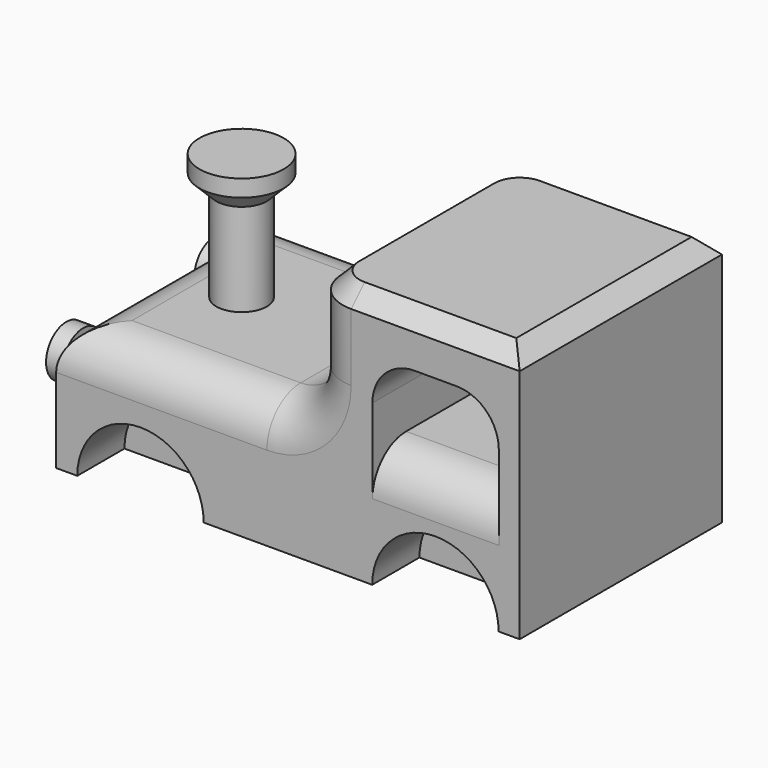
from build123d import *

# Parameters (mm, degrees)
F0_W      = 55
F0_H      = 30
F1_DEPTH  = 30
F2_W      = 30
F2_H      = 15
F3_DEPTH  = 30.001
F5_DEPTH  = 7
F6_F1_R   = 5
F6_F2_R   = 5
F7_SIZE   = 2
F9_DEPTH  = 30.001
F10_R     = 5
F12_DEPTH = 2
F13_R     = 3
F14_DEPTH = 15
F15_R     = 5
F15_R_2   = 3
F16_DEPTH = 4
F17_SIZE  = 1.99999


# Not quite as in the source:
# - a fillet or chamfer is up to 0.001 mm smaller than in the source, because OpenCascade refuses the exact size
# - a pattern or mirror of a feature is missing from the dataset's text; its kind, count and spacing are read off the source's solid


with BuildPart() as f1:
    # F0 (on Top) → F1 (new body)
    with BuildSketch(Plane.XY):
        Rectangle(F0_W, F0_H)
    extrude(amount=F1_DEPTH)

    # F2 (on face) → F3 (cut, through all)
    with BuildSketch(Plane.XZ.offset(15)):
        with Locations((-12.5, 22.5)):
            Rectangle(F2_W, F2_H)
    extrude(amount=-F3_DEPTH, mode=Mode.SUBTRACT)

    # F4 (on face) → F5 (cut)
    with BuildSketch(Plane.XZ.offset(15)):
        with BuildLine():
            Line((-25, 0), (-10, 0))
            ThreePointArc((-10, 0), (-17.5, 7.5), (-25, 0))
        make_face()
        with BuildLine():
            ThreePointArc((25, 0), (17.5, 7.5), (10, 0))
            Line((10, 0), (25, 0))
        make_face()
    f5 = extrude(amount=-F5_DEPTH, mode=Mode.SUBTRACT)

    # F5_copies: F5 across plane
    add(f5.mirror(Plane.ZX), mode=Mode.SUBTRACT)

    # F6: fillet of radius 5 on 4 edges, made by hand

    # F6_f1
    f6_f1_edges = [f1.edges().sort_by_distance(p)[0] for p in [
        (2.5, 0, 15),
    ]]
    fillet(f6_f1_edges, radius=F6_F1_R)

    # F6_f2
    f6_f2_edges = [f1.edges().sort_by_distance(p)[0] for p in [
        (-15, -15, 15),
        (-15, 15, 15),
        (-27.5, 0, 15),
        (1.0355339059, 15, 16.4644660941),
        (1.0355339059, -15, 16.4644660941),
    ]]
    fillet(f6_f2_edges, radius=F6_F2_R)

    # F7
    f7_edges = [f1.edges().sort_by_distance(p)[0] for p in [
        (17.5, -15, 30),
        (3.964466, -13.535534, 30),
        (27.5, 0, 30),
        (2.5, 0, 30),
        (17.5, 15, 30),
        (3.964466, 13.535534, 30),
    ]]
    chamfer(f7_edges, length=F7_SIZE)

    # F8 (on face) → F9 (cut, through all)
    with BuildSketch(Plane.XZ.offset(15)):
        with BuildLine():
            Line((20.0235929713, 24), (15.0235929713, 24))
            ThreePointArc((15.0235929713, 24), (11.4880590653, 22.5355339059), (10.0235929713, 19))
            Line((10.0235929713, 19), (10.0235929713, 14))
            Line((10.0235929713, 14), (25.0235929713, 14))
            Line((25.0235929713, 14), (25.0235929713, 19))
            ThreePointArc((25.0235929713, 19), (23.5591268772, 22.5355339059), (20.0235929713, 24))
        make_face()
    extrude(amount=-F9_DEPTH, mode=Mode.SUBTRACT)

    # F10
    f10_edges = [f1.edges().sort_by_distance(p)[0] for p in [
        (17.523593, -15, 14),
        (17.523593, 15, 14),
    ]]
    fillet(f10_edges, radius=F10_R)

    # F11 (on face) → F12 (join)
    with BuildSketch(Plane(origin=(-27.5, 0, 0), x_dir=(0, -1, 0), z_dir=(-1, 0, 0))):
        with BuildLine():
            Line((-14, 10), (-8, 10))
            ThreePointArc((-8, 10), (-11, 13), (-14, 10))
        make_face()
        with BuildLine():
            ThreePointArc((-14, 10), (-11, 7), (-8, 10))
            Line((-8, 10), (-14, 10))
        make_face()
        with BuildLine():
            Line((14, 10), (8, 10))
            ThreePointArc((8, 10), (11, 7), (14, 10))
        make_face()
        with BuildLine():
            ThreePointArc((14, 10), (11, 13), (8, 10))
            Line((8, 10), (14, 10))
        make_face()
    extrude(amount=F12_DEPTH)

    # F13 (on face) → F14 (join)
    with BuildSketch(Plane.XY.offset(15)):
        with Locations((-17.5, 0)):
            Circle(F13_R)
    extrude(amount=F14_DEPTH)

    # F15 (on face) → F16 (join)
    with BuildSketch(Plane.XY.offset(30)):
        with Locations((-17.5, 0)):
            Circle(F15_R)
        with Locations((-17.5, 0)):
            Circle(F15_R_2, mode=Mode.SUBTRACT)
    extrude(amount=-F16_DEPTH)

    # F17 (size 2 in the source; OpenCascade refuses exactly that, so slightly less here)
    f17_edges = [f1.edges().sort_by_distance(p)[0] for p in [
        (-22.5, 0, 26),
    ]]
    chamfer(f17_edges, length=F17_SIZE)


solid = f1.part
